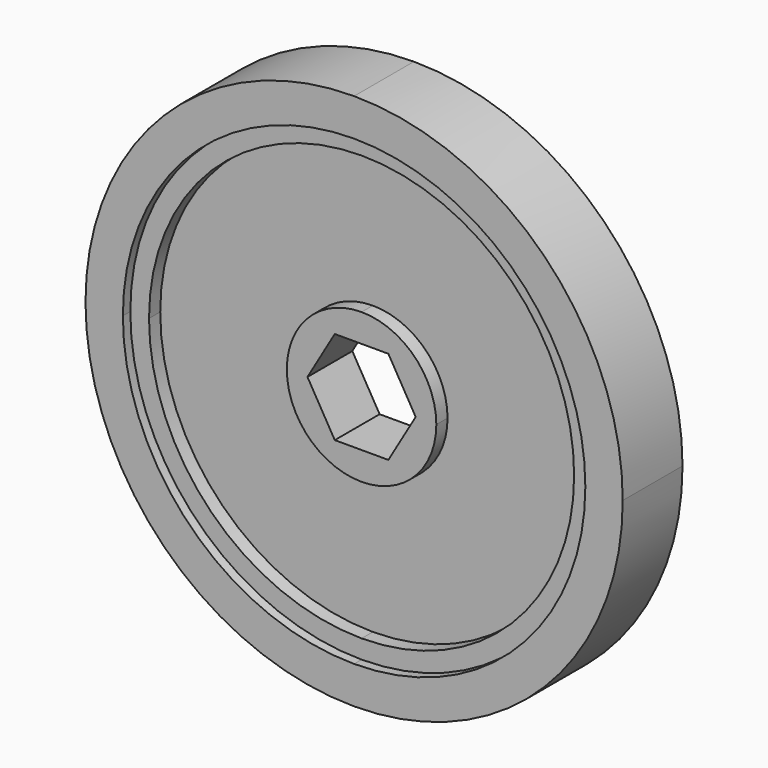
from build123d import *

# Parameters (mm, degrees)
F1_DEPTH = 5.08
F2_DEPTH = 3.81
F3_DEPTH = 1.905


with BuildPart() as f1:
    # F0 (on Front) → F1 (new body, symmetric)
    with BuildSketch(Plane.XZ):
        with BuildLine():
            ThreePointArc((0, 31.4325), (22.226134, 22.226134), (31.4325, 0))
            Line((31.4325, 0), (36.5125, 0))
            ThreePointArc((36.5125, 0), (25.818236, 25.818236), (0, 36.5125))
            Line((0, 36.5125), (0, 31.4325))
        make_face()
        with BuildLine():
            Line((0, -36.5125), (0, -31.4325))
            ThreePointArc((0, -31.4325), (-22.226134, -22.226134), (-31.4325, 0))
            Line((-31.4325, 0), (-36.5125, 0))
            ThreePointArc((-36.5125, 0), (-25.818236, -25.818236), (0, -36.5125))
        make_face()
        with BuildLine():
            Line((36.5125, 0), (31.4325, 0))
            ThreePointArc((31.4325, 0), (22.226134, -22.226134), (0, -31.4325))
            Line((0, -31.4325), (0, -36.5125))
            ThreePointArc((0, -36.5125), (25.818236, -25.818236), (36.5125, 0))
        make_face()
        with BuildLine():
            ThreePointArc((-31.4325, 0), (-22.226134, 22.226134), (0, 31.4325))
            Line((0, 31.4325), (0, 36.5125))
            ThreePointArc((0, 36.5125), (-25.818236, 25.818236), (-36.5125, 0))
            Line((-36.5125, 0), (-31.4325, 0))
        make_face()
    extrude(amount=F1_DEPTH, both=True)

    # F0 (on Front) → F2, piece 2 (join, symmetric)
    with BuildSketch(Plane.XZ):
        with BuildLine():
            Line((0, 28.8925), (0, 31.4325))
            ThreePointArc((0, 31.4325), (-22.226134, 22.226134), (-31.4325, 0))
            Line((-31.4325, 0), (-28.8925, 0))
            ThreePointArc((-28.8925, 0), (-20.430083, 20.430083), (0, 28.8925))
        make_face()
        with BuildLine():
            Line((28.8925, 0), (31.4325, 0))
            ThreePointArc((31.4325, 0), (22.226134, 22.226134), (0, 31.4325))
            Line((0, 31.4325), (0, 28.8925))
            ThreePointArc((0, 28.8925), (20.430083, 20.430083), (28.8925, 0))
        make_face()
        with BuildLine():
            ThreePointArc((0, -31.4325), (22.226134, -22.226134), (31.4325, 0))
            Line((31.4325, 0), (28.8925, 0))
            ThreePointArc((28.8925, 0), (20.430083, -20.430083), (0, -28.8925))
            Line((0, -28.8925), (0, -31.4325))
        make_face()
        with BuildLine():
            ThreePointArc((-31.4325, 0), (-22.226134, -22.226134), (0, -31.4325))
            Line((0, -31.4325), (0, -28.8925))
            ThreePointArc((0, -28.8925), (-20.430083, -20.430083), (-28.8925, 0))
            Line((-28.8925, 0), (-31.4325, 0))
        make_face()
    extrude(amount=F2_DEPTH, both=True)


with BuildPart() as f2:
    # F0 (on Front) → F2 (new body, symmetric)
    with BuildSketch(Plane.XZ):
        with BuildLine():
            Line((0, 6.35), (0, 10.16))
            ThreePointArc((0, 10.16), (-7.184205, 7.184205), (-10.16, 0))
            Line((-10.16, 0), (-7.354874, 0))
            Line((-7.354874, 0), (-3.643854, 6.35))
            Line((-3.643854, 6.35), (0, 6.35))
        make_face()
        with BuildLine():
            Line((7.354874, 0), (10.16, 0))
            ThreePointArc((10.16, 0), (7.184205, 7.184205), (0, 10.16))
            Line((0, 10.16), (0, 6.35))
            Line((0, 6.35), (3.643854, 6.35))
            Line((3.643854, 6.35), (7.354874, 0))
        make_face()
        with BuildLine():
            ThreePointArc((0, -10.16), (7.184205, -7.184205), (10.16, 0))
            Line((10.16, 0), (7.354874, 0))
            Line((7.354874, 0), (3.643854, -6.35))
            Line((3.643854, -6.35), (0, -6.35))
            Line((0, -6.35), (0, -10.16))
        make_face()
        with BuildLine():
            ThreePointArc((-10.16, 0), (-7.184205, -7.184205), (0, -10.16))
            Line((0, -10.16), (0, -6.35))
            Line((0, -6.35), (-3.643854, -6.35))
            Line((-3.643854, -6.35), (-7.354874, 0))
            Line((-7.354874, 0), (-10.16, 0))
        make_face()
    extrude(amount=F2_DEPTH, both=True)


with BuildPart() as f3:
    # F0 (on Front) → F3 (new body, symmetric)
    with BuildSketch(Plane.XZ):
        with BuildLine():
            Line((10.16, 0), (28.8925, 0))
            ThreePointArc((28.8925, 0), (20.430083, 20.430083), (0, 28.8925))
            Line((0, 28.8925), (0, 10.16))
            ThreePointArc((0, 10.16), (7.184205, 7.184205), (10.16, 0))
        make_face()
        with BuildLine():
            ThreePointArc((0, -28.8925), (20.430083, -20.430083), (28.8925, 0))
            Line((28.8925, 0), (10.16, 0))
            ThreePointArc((10.16, 0), (7.184205, -7.184205), (0, -10.16))
            Line((0, -10.16), (0, -28.8925))
        make_face()
        with BuildLine():
            ThreePointArc((-28.8925, 0), (-20.430083, -20.430083), (0, -28.8925))
            Line((0, -28.8925), (0, -10.16))
            ThreePointArc((0, -10.16), (-7.184205, -7.184205), (-10.16, 0))
            Line((-10.16, 0), (-28.8925, 0))
        make_face()
        with BuildLine():
            Line((0, 10.16), (0, 28.8925))
            ThreePointArc((0, 28.8925), (-20.430083, 20.430083), (-28.8925, 0))
            Line((-28.8925, 0), (-10.16, 0))
            ThreePointArc((-10.16, 0), (-7.184205, 7.184205), (0, 10.16))
        make_face()
    extrude(amount=F3_DEPTH, both=True)


solid = Compound([f1.part, f2.part, f3.part])
